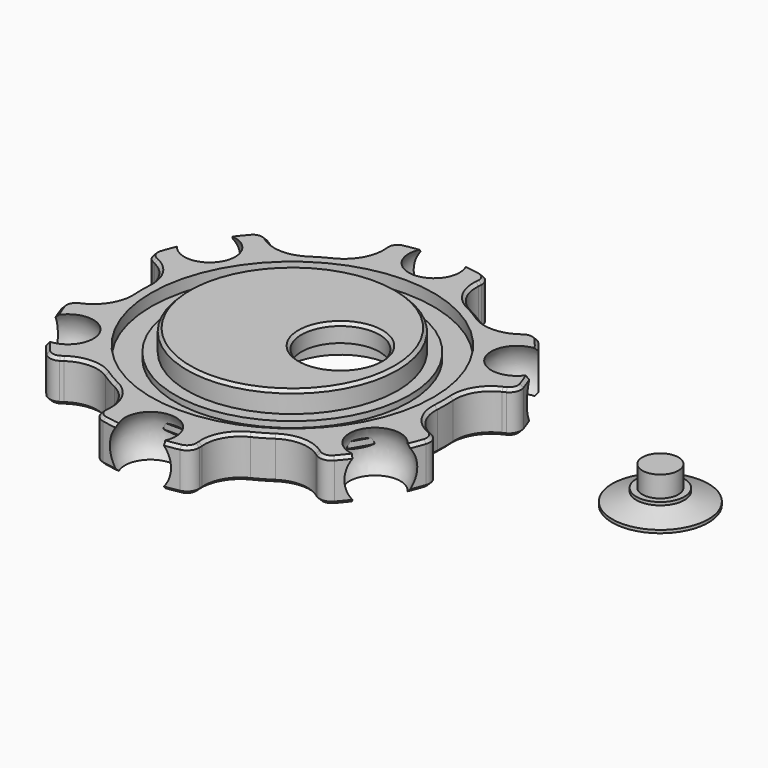
from build123d import *

# Parameters (mm, degrees)
F0_R          = 23.5
F1_DEPTH      = 3.5
F1_DEPTH_BACK = 3.5
F2_R          = 6
F3_R          = 2
F4_SIZE       = 0.5
F5_COUNT      = 6
F13_R         = 24.5
F13_R_2       = 19.5
F14_DEPTH     = 1.5
F13_R_3       = 17.5
F15_DEPTH     = 2.5
F13_R_4       = 9
F13_R_5       = 6.5
F16_DEPTH     = 6
F17_DEPTH     = 3
F18_SIZE      = 0.5


with BuildPart() as f1:
    # F0 (on Top) → F1 (new body, two sides)
    with BuildSketch(Plane.XY) as f1_sk:
        with BuildLine():
            ThreePointArc((-7.8540430234, 31.0211864407), (-7.794489988, 27.698354689), (-6.3898080295, 24.686440678))
            ThreePointArc((-6.3898080295, 24.686440678), (0, -25.5), (6.3898080295, 24.686440678))
            ThreePointArc((6.3898080295, 24.686440678), (7.794489988, 27.698354689), (7.8540430234, 31.0211864407))
            ThreePointArc((7.8540430234, 31.0211864407), (5.2200485514, 31.5713650817), (2.5491435269, 31.8983050847))
            ThreePointArc((2.5491435269, 31.8983050847), (0, 26), (-2.5491435269, 31.8983050847))
            ThreePointArc((-2.5491435269, 31.8983050847), (-5.2200485514, 31.5713650817), (-7.8540430234, 31.0211864407))
        make_face()
        Circle(F0_R, mode=Mode.SUBTRACT)
    extrude(amount=F1_DEPTH)
    extrude(f1_sk.sketch, amount=-F1_DEPTH_BACK)

    # F2
    f2_edges = [f1.edges().sort_by_distance(p)[0] for p in [
        (-6.389808, 24.686441, 0),
        (6.389808, 24.686441, 0),
    ]]
    fillet(f2_edges, radius=F2_R)

    # F3
    f3_edges = [f1.edges().sort_by_distance(p)[0] for p in [
        (-7.854043, 31.021186, 0),
        (7.854043, 31.021186, 0),
    ]]
    fillet(f3_edges, radius=F3_R)

    # F4
    f4_edges = [f1.edges().sort_by_distance(p)[0] for p in [
        (-4.482353, 31.684515, -3.5),
        (-8.710943, 25.310083, -3.5),
        (4.482353, 31.684515, 3.5),
        (-7.988476, 29.070746, -3.5),
        (-7.559345, 30.645278, -3.5),
        (0, -25.5, -3.5),
        (8.710943, 25.310083, -3.5),
        (4.482353, 31.684515, -3.5),
        (7.988476, 29.070746, -3.5),
        (7.559345, 30.645278, -3.5),
        (-7.988476, 29.070746, 3.5),
        (-7.559345, 30.645278, 3.5),
        (-8.710943, 25.310083, 3.5),
        (-4.482353, 31.684515, 3.5),
        (0, -25.5, 3.5),
        (8.710943, 25.310083, 3.5),
        (7.988476, 29.070746, 3.5),
        (7.559345, 30.645278, 3.5),
    ]]
    chamfer(f4_edges, length=F4_SIZE)

    # F5: F1 ×6 about axis
    f5_axis = Axis((0, 0, 0), (0, 0, 1))


with BuildPart() as f1_1:
    add(f1.part)
    for i in range(1, F5_COUNT):
        add(f1.part.rotate(f5_axis, i * 360 / F5_COUNT))

    # F6 (on Top) → F7 (revolve, cut)
    with BuildSketch(Plane.XY):
        with BuildLine():
            Line((5.5, 29.5), (-5.5, 29.5))
            ThreePointArc((-5.5, 29.5), (0, 24), (5.5, 29.5))
        make_face()
    revolve(axis=Axis((0, 29.5, 0), (1, 0, 0)), mode=Mode.SUBTRACT)

    # F6 (on Top) → F8 (revolve, cut)
    with BuildSketch(Plane.XY):
        with BuildLine():
            Line((-22.7977494116, 19.5131397208), (-28.2977494116, 9.9868602792))
            ThreePointArc((-28.2977494116, 9.9868602792), (-20.7846096908, 12), (-22.7977494116, 19.5131397208))
        make_face()
    revolve(axis=Axis((-25.5477494116, 14.75, 0), (0.5, 0.8660254038, 0)), mode=Mode.SUBTRACT)

    # F6 (on Top) → F9 (revolve, cut)
    with BuildSketch(Plane.XY):
        with BuildLine():
            Line((-28.2977494116, -9.9868602792), (-22.7977494116, -19.5131397208))
            ThreePointArc((-22.7977494116, -19.5131397208), (-20.7846096908, -12), (-28.2977494116, -9.9868602792))
        make_face()
    revolve(axis=Axis((-25.5477494116, -14.75, 0), (-0.5, 0.8660254038, 0)), mode=Mode.SUBTRACT)

    # F6 (on Top) → F10 (revolve, cut)
    with BuildSketch(Plane.XY):
        with BuildLine():
            Line((-5.5, -29.5), (5.5, -29.5))
            ThreePointArc((5.5, -29.5), (0, -24), (-5.5, -29.5))
        make_face()
    revolve(axis=Axis((0, -29.5, 0), (-1, 0, 0)), mode=Mode.SUBTRACT)

    # F6 (on Top) → F11 (revolve, cut)
    with BuildSketch(Plane.XY):
        with BuildLine():
            Line((22.7977494116, -19.5131397208), (28.2977494116, -9.9868602792))
            ThreePointArc((28.2977494116, -9.9868602792), (20.7846096908, -12), (22.7977494116, -19.5131397208))
        make_face()
    revolve(axis=Axis((25.5477494116, -14.75, 0), (-0.5, -0.8660254038, 0)), mode=Mode.SUBTRACT)

    # F6 (on Top) → F12 (revolve, cut)
    with BuildSketch(Plane.XY):
        with BuildLine():
            Line((28.2977494116, 9.9868602792), (22.7977494116, 19.5131397208))
            ThreePointArc((22.7977494116, 19.5131397208), (20.7846096908, 12), (28.2977494116, 9.9868602792))
        make_face()
    revolve(axis=Axis((25.5477494116, 14.75, 0), (0.5, -0.8660254038, 0)), mode=Mode.SUBTRACT)


with BuildPart() as f14:
    # F13 (on Top) → F14 (new body)
    with BuildSketch(Plane.XY):
        Circle(F13_R)
        Circle(F13_R_2, mode=Mode.SUBTRACT)
    extrude(amount=F14_DEPTH)

    # F13 (on Top) → F15 (join)
    with BuildSketch(Plane.XY):
        Circle(F13_R_2)
        Circle(F13_R_3, mode=Mode.SUBTRACT)
    extrude(amount=F15_DEPTH)

    # F13 (on Top) → F16 (join)
    with BuildSketch(Plane.XY):
        Circle(F13_R_3)
        with Locations((8, 0)):
            Circle(F13_R_4, mode=Mode.SUBTRACT)
        with Locations((8, 0)):
            Circle(F13_R_4)
        with Locations((8, 0)):
            Circle(F13_R_5, mode=Mode.SUBTRACT)
    extrude(amount=F16_DEPTH)

    # F13 (on Top) → F17 (cut)
    with BuildSketch(Plane.XY):
        with Locations((8, 0)):
            Circle(F13_R_4)
        with Locations((8, 0)):
            Circle(F13_R_5, mode=Mode.SUBTRACT)
    extrude(amount=F17_DEPTH, mode=Mode.SUBTRACT)

    # F18
    f18_edges = [f14.edges().sort_by_distance(p)[0] for p in [
        (-17.5, 0, 6),
        (1.5, 0, 6),
        (-24.5, 0, 0),
    ]]
    chamfer(f18_edges, length=F18_SIZE)


with BuildPart() as f20:
    # F19 (on Front) → F20 (revolve)
    with BuildSketch(Plane.XZ):
        Polygon((61.2371124625, 0), (61.2371124625, 6), (58.2371124625, 6), (58.2371124625, 2.5), (57.2371124625, 2.5), (57.2371124625, 2), (53.2371124625, 0.5), (53.2371124625, 0), align=None)
    revolve(axis=Axis((61.2371124625, 0, 3), (0, 0, -1)))


solid = Compound([f1_1.part, f14.part, f20.part])
